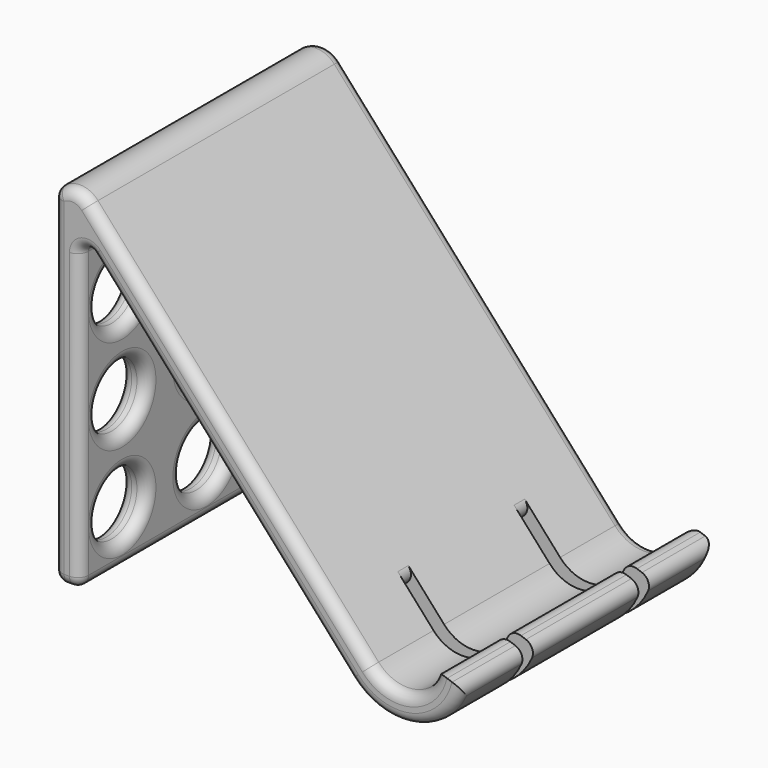
from build123d import *

# Parameters (mm, degrees)
F1_DEPTH = 76.2
F2_R     = 7.62
F3_DEPTH = 6.35
F4_W     = 3.175
F4_H     = 15.24
F5_DEPTH = 76.2
F6_R     = 2.53999
F7_R     = 2.54


# Not quite as in the source:
# - a fillet or chamfer is up to 0.001 mm smaller than in the source, because OpenCascade refuses the exact size


with BuildPart() as f1:
    # F0 (on Front) → F1 (new body)
    with BuildSketch(Plane.XZ):
        with BuildLine():
            Line((28.7842985747, -26.5391112355), (-38.797929834, 49.323939081))
            ThreePointArc((-38.797929834, 49.323939081), (-43.1274730528, 51.2653507655), (-47.4570162716, 49.323939081))
            Line((-47.4570162716, 49.323939081), (-47.4570162716, -33.3967016697))
            Line((-47.4570162716, -33.3967016697), (-41.1070162716, -33.3967016697))
            Line((-41.1070162716, -33.3967016697), (-41.1070162716, 37.7979404016))
            ThreePointArc((-41.1070162716, 37.7979404016), (-39.9856080884, 39.4249731546), (-38.0660023348, 38.956032174))
            Line((-38.0660023348, 38.956032174), (24.0428579299, -30.763000511))
            ThreePointArc((24.0428579299, -30.763000511), (39.4296194954, -35.5416750714), (50.8525124736, -24.179207116))
            Line((50.8525124736, -24.179207116), (44.8236542685, -22.031940877))
            ThreePointArc((44.8236542685, -22.031940877), (38.2121629119, -29.2967420087), (28.7842985747, -26.5391112355))
        make_face()
    extrude(amount=F1_DEPTH)

    # F2 (on face) → F3 (cut)
    with BuildSketch(Plane(origin=(-47.4570162716, 0, 0), x_dir=(0, -1, 0), z_dir=(-1, 0, 0))):
        with Locations((12.7, -20.5108800562)):
            Circle(F2_R)
        with Locations((38.1, -20.5108800562)):
            Circle(F2_R)
        with Locations((63.5, -20.5108800562)):
            Circle(F2_R)
        with Locations((12.7, 2.3491199438)):
            Circle(F2_R)
        with Locations((38.1, 2.3491199438)):
            Circle(F2_R)
        with Locations((63.5, 2.3491199438)):
            Circle(F2_R)
        with Locations((12.7, 25.2091199438)):
            Circle(F2_R)
        with Locations((38.1, 25.2091199438)):
            Circle(F2_R)
        with Locations((63.5, 25.2091199438)):
            Circle(F2_R)
    extrude(amount=-F3_DEPTH, mode=Mode.SUBTRACT)

    # F4 (on Right) → F5 (cut)
    with BuildSketch(Plane.YZ):
        with Locations((-55.5625, -28.7159914046)):
            Rectangle(F4_W, F4_H)
        with Locations((-20.6375, -28.8014974874)):
            Rectangle(F4_W, F4_H)
    extrude(amount=F5_DEPTH, mode=Mode.SUBTRACT)

    # F6 (radius 2.54 in the source; OpenCascade refuses exactly that, so slightly less here)
    f6_edges = [f1.edges().sort_by_distance(p)[0] for p in [
        (-41.107016, -38.1, -33.396702),
        (-47.457016, -38.1, -33.396702),
        (-44.282016, 0, -33.396702),
        (-44.282016, -76.2, -33.396702),
        (-41.107016, 0, 2.200619),
        (-47.457016, 0, 7.963619),
        (-47.457016, -38.1, 49.323939),
        (-47.457016, -76.2, 7.963619),
        (-41.107016, -76.2, 2.200619),
        (-43.127473, 0, 51.265351),
        (-5.006816, 0, 11.392414),
        (-43.127473, -76.2, 51.265351),
        (50.852512, -38.1, -24.179207),
        (44.823654, -38.1, -22.031941),
        (50.852512, -9.525, -24.179207),
        (44.823654, -9.525, -22.031941),
        (50.852512, -66.675, -24.179207),
        (44.823654, -66.675, -22.031941),
        (-41.107016, -5.08, 2.34912),
        (-41.107016, -5.08, 25.20912),
        (-41.107016, -5.08, -20.51088),
        (-41.107016, -30.48, -20.51088),
        (-41.107016, -30.48, 2.34912),
        (-41.107016, -30.48, 25.20912),
        (-41.107016, -55.88, -20.51088),
        (-41.107016, -55.88, 2.34912),
        (-41.107016, -55.88, 25.20912),
        (-47.457016, -5.08, 25.20912),
        (-47.457016, -30.48, 25.20912),
        (-47.457016, -55.88, 25.20912),
        (-47.457016, -55.88, 2.34912),
        (-47.457016, -30.48, 2.34912),
        (-47.457016, -5.08, 2.34912),
        (-47.457016, -5.08, -20.51088),
        (-47.457016, -30.48, -20.51088),
        (-47.457016, -55.88, -20.51088),
    ]]
    fillet(f6_edges, radius=F6_R)

    # F7
    f7_edges = [f1.edges().sort_by_distance(p)[0] for p in [
        (23.935322, -55.5625, -21.095991),
        (24.011494, -20.6375, -21.181497),
    ]]
    fillet(f7_edges, radius=F7_R)


solid = f1.part
